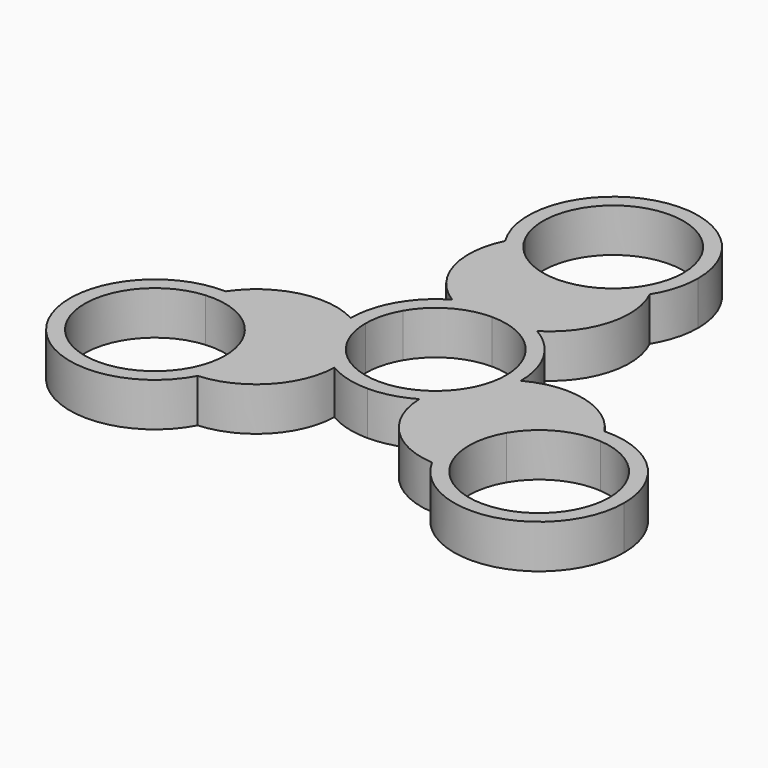
from build123d import *

# Parameters (mm, degrees)
F1_DEPTH = 5.9


with BuildPart() as f1:
    # F0 (on Top) → F1 (new body)
    with BuildSketch(Plane.XY):
        with BuildLine():
            Line((11.5, 0), (9.5, 0))
            ThreePointArc((9.5, 0), (9.1762953497, -2.4587809285), (8.227241336, -4.75))
            Line((8.227241336, -4.75), (9.9592921435, -5.75))
            ThreePointArc((9.9592921435, -5.75), (11.1081470023, -2.9764190187), (11.5, 0))
        make_face()
        with BuildLine():
            ThreePointArc((8.227241336, 4.75), (9.1762953497, 2.4587809285), (9.5, 0))
            Line((9.5, 0), (11.5, 0))
            ThreePointArc((11.5, 0), (11.1081470023, 2.9764190187), (9.9592921435, 5.75))
            Line((9.9592921435, 5.75), (8.227241336, 4.75))
        make_face()
        with BuildLine():
            ThreePointArc((0, 9.5), (4.75, 8.227241336), (8.227241336, 4.75))
            Line((8.227241336, 4.75), (9.9592921435, 5.75))
            ThreePointArc((9.9592921435, 5.75), (8.1317279836, 8.1317279836), (5.75, 9.9592921435))
            ThreePointArc((5.75, 9.9592921435), (2.9764190187, 11.1081470023), (0, 11.5))
            Line((0, 11.5), (0, 9.5))
        make_face()
        with BuildLine():
            Line((9.9592921435, -5.75), (8.227241336, -4.75))
            ThreePointArc((8.227241336, -4.75), (4.75, -8.227241336), (0, -9.5))
            Line((0, -9.5), (0, -11.5))
            ThreePointArc((0, -11.5), (2.9764190187, -11.1081470023), (5.75, -9.9592921435))
            ThreePointArc((5.75, -9.9592921435), (8.1317279836, -8.1317279836), (9.9592921435, -5.75))
        make_face()
        with BuildLine():
            Line((21.7644823154, 0), (11.5, 0))
            ThreePointArc((11.5, 0), (11.1081470023, -2.9764190187), (9.9592921435, -5.75))
            Line((9.9592921435, -5.75), (16.02146997, -9.25))
            ThreePointArc((16.02146997, -9.25), (20.0781480078, -5.1303927779), (25.6267837466, -3.5054491468))
            ThreePointArc((25.6267837466, -3.5054491468), (23.9098470955, -1.5167036662), (21.7644823154, 0))
        make_face()
        with BuildLine():
            ThreePointArc((21.7644823154, 0), (16.6322411577, 1.2934670156), (11.5, 0))
            Line((11.5, 0), (21.7644823154, 0))
        make_face()
        with BuildLine():
            ThreePointArc((-8.227241336, 4.75), (-4.75, 8.227241336), (0, 9.5))
            Line((0, 9.5), (0, 11.5))
            ThreePointArc((0, 11.5), (-2.9764190187, 11.1081470023), (-5.75, 9.9592921435))
            ThreePointArc((-5.75, 9.9592921435), (-8.1317279836, 8.1317279836), (-9.9592921435, 5.75))
            Line((-9.9592921435, 5.75), (-8.227241336, 4.75))
        make_face()
        with BuildLine():
            Line((0, -11.5), (0, -9.5))
            ThreePointArc((0, -9.5), (-4.75, -8.227241336), (-8.227241336, -4.75))
            Line((-8.227241336, -4.75), (-9.9592921435, -5.75))
            ThreePointArc((-9.9592921435, -5.75), (-8.1317279836, -8.1317279836), (-5.75, -9.9592921435))
            ThreePointArc((-5.75, -9.9592921435), (-2.9764190187, -11.1081470023), (0, -11.5))
        make_face()
        with BuildLine():
            Line((16.02146997, -9.25), (9.9592921435, -5.75))
            ThreePointArc((9.9592921435, -5.75), (8.1317279836, -8.1317279836), (5.75, -9.9592921435))
            ThreePointArc((5.75, -9.9592921435), (8.7759533757, -17.1498563505), (15.8491998862, -20.4407211685))
            ThreePointArc((15.8491998862, -20.4407211685), (14.4821244809, -14.8229898467), (16.02146997, -9.25))
        make_face()
        with BuildLine():
            Line((-9.9592921435, -5.75), (-8.227241336, -4.75))
            ThreePointArc((-8.227241336, -4.75), (-9.1762953497, -2.4587809285), (-9.5, 0))
            Line((-9.5, 0), (-11.5, 0))
            ThreePointArc((-11.5, 0), (-11.1081470023, -2.9764190187), (-9.9592921435, -5.75))
        make_face()
        with BuildLine():
            Line((-11.5, 0), (-9.5, 0))
            ThreePointArc((-9.5, 0), (-9.1762953497, 2.4587809285), (-8.227241336, 4.75))
            Line((-8.227241336, 4.75), (-9.9592921435, 5.75))
            ThreePointArc((-9.9592921435, 5.75), (-11.1081470023, 2.9764190187), (-11.5, 0))
        make_face()
        with BuildLine():
            Line((0, 18.5), (0, 11.5))
            ThreePointArc((0, 11.5), (2.9764190187, 11.1081470023), (5.75, 9.9592921435))
            ThreePointArc((5.75, 9.9592921435), (10.464234583, 16.1751267411), (9.7775838605, 23.9461703153))
            ThreePointArc((9.7775838605, 23.9461703153), (5.5960235268, 19.9533826246), (0, 18.5))
        make_face()
        with BuildLine():
            ThreePointArc((-5.75, 9.9592921435), (-2.9764190187, 11.1081470023), (0, 11.5))
            Line((0, 11.5), (0, 18.5))
            ThreePointArc((0, 18.5), (-5.5960235268, 19.9533826246), (-9.7775838605, 23.9461703153))
            ThreePointArc((-9.7775838605, 23.9461703153), (-10.464234583, 16.1751267411), (-5.75, 9.9592921435))
        make_face()
        with BuildLine():
            ThreePointArc((25.6267837466, -3.5054491468), (20.0781480078, -5.1303927779), (16.02146997, -9.25))
            Line((16.02146997, -9.25), (17.7535207776, -10.25))
            ThreePointArc((17.7535207776, -10.25), (21.5421151907, -6.6006897013), (26.6916116991, -5.5266324432))
            ThreePointArc((26.6916116991, -5.5266324432), (26.212648084, -4.4878813308), (25.6267837466, -3.5054491468))
        make_face()
        with BuildLine():
            Line((17.7535207776, -10.25), (16.02146997, -9.25))
            ThreePointArc((16.02146997, -9.25), (14.4821244809, -14.8229898467), (15.8491998862, -20.4407211685))
            ThreePointArc((15.8491998862, -20.4407211685), (16.9929432837, -20.4568784758), (18.1320099427, -20.3522975778))
            ThreePointArc((18.1320099427, -20.3522975778), (16.4874225591, -15.3556741558), (17.7535207776, -10.25))
        make_face()
        with BuildLine():
            Line((-16.02146997, -9.25), (-9.9592921435, -5.75))
            ThreePointArc((-9.9592921435, -5.75), (-11.1081470023, -2.9764190187), (-11.5, 0))
            Line((-11.5, 0), (-21.7644823154, 0))
            ThreePointArc((-21.7644823154, 0), (-23.9098470955, -1.5167036662), (-25.6267837466, -3.5054491468))
            ThreePointArc((-25.6267837466, -3.5054491468), (-20.0781480078, -5.1303927779), (-16.02146997, -9.25))
        make_face()
        with BuildLine():
            ThreePointArc((-5.75, -9.9592921435), (-8.1317279836, -8.1317279836), (-9.9592921435, -5.75))
            Line((-9.9592921435, -5.75), (-16.02146997, -9.25))
            ThreePointArc((-16.02146997, -9.25), (-14.8726151112, -12.0235809813), (-14.4807621135, -15))
            ThreePointArc((-14.4807621135, -15), (-14.8281174582, -17.8050877335), (-15.8491998862, -20.4407211685))
            ThreePointArc((-15.8491998862, -20.4407211685), (-8.7759533757, -17.1498563505), (-5.75, -9.9592921435))
        make_face()
        with BuildLine():
            Line((-21.7644823154, 0), (-11.5, 0))
            ThreePointArc((-11.5, 0), (-16.6322411577, 1.2934670156), (-21.7644823154, 0))
        make_face()
        with BuildLine():
            ThreePointArc((37.4807621135, -15), (33.9863616782, -6.7440702759), (25.6267837466, -3.5054491468))
            ThreePointArc((25.6267837466, -3.5054491468), (26.212648084, -4.4878813308), (26.6916116991, -5.5266324432))
            ThreePointArc((26.6916116991, -5.5266324432), (32.945066496, -8.5386948324), (35.4807621135, -15))
            ThreePointArc((35.4807621135, -15), (28.7813740446, -24.077806608), (18.1320099427, -20.3522975778))
            ThreePointArc((18.1320099427, -20.3522975778), (16.9929432837, -20.4568784758), (15.8491998862, -20.4407211685))
            ThreePointArc((15.8491998862, -20.4407211685), (28.785849847, -26.1526446553), (37.4807621135, -15))
        make_face()
        with BuildLine():
            ThreePointArc((-9.7775838605, 23.9461703153), (-5.5960235268, 19.9533826246), (0, 18.5))
            Line((0, 18.5), (0, 20.5))
            ThreePointArc((0, 20.5), (-5.0546926316, 21.956363857), (-8.5596017564, 25.8789300209))
            ThreePointArc((-8.5596017564, 25.8789300209), (-9.2197048003, 24.9447598066), (-9.7775838605, 23.9461703153))
        make_face()
        with BuildLine():
            Line((0, 20.5), (0, 18.5))
            ThreePointArc((0, 18.5), (5.5960235268, 19.9533826246), (9.7775838605, 23.9461703153))
            ThreePointArc((9.7775838605, 23.9461703153), (9.2197048003, 24.9447598066), (8.5596017564, 25.8789300209))
            ThreePointArc((8.5596017564, 25.8789300209), (5.0546926316, 21.956363857), (0, 20.5))
        make_face()
        with BuildLine():
            ThreePointArc((8.5596017564, 25.8789300209), (9.2197048003, 24.9447598066), (9.7775838605, 23.9461703153))
            ThreePointArc((9.7775838605, 23.9461703153), (11.0610174576, 26.8529549094), (11.5, 30))
            ThreePointArc((11.5, 30), (-3.1470450906, 41.0610174576), (-9.7775838605, 23.9461703153))
            ThreePointArc((-9.7775838605, 23.9461703153), (-9.2197048003, 24.9447598066), (-8.5596017564, 25.8789300209))
            ThreePointArc((-8.5596017564, 25.8789300209), (-2.1135022255, 39.2619170987), (9.5, 30))
            ThreePointArc((9.5, 30), (9.2619170987, 27.8864977745), (8.5596017564, 25.8789300209))
        make_face()
        with BuildLine():
            ThreePointArc((-14.4807621135, -15), (-14.8726151112, -12.0235809813), (-16.02146997, -9.25))
            Line((-16.02146997, -9.25), (-17.7535207776, -10.25))
            ThreePointArc((-17.7535207776, -10.25), (-16.8044667638, -12.5412190715), (-16.4807621135, -15))
            ThreePointArc((-16.4807621135, -15), (-16.9029555056, -17.8006119311), (-18.1320099427, -20.3522975778))
            ThreePointArc((-18.1320099427, -20.3522975778), (-16.9929432837, -20.4568784758), (-15.8491998862, -20.4407211685))
            ThreePointArc((-15.8491998862, -20.4407211685), (-14.8281174582, -17.8050877335), (-14.4807621135, -15))
        make_face()
        with BuildLine():
            Line((-17.7535207776, -10.25), (-16.02146997, -9.25))
            ThreePointArc((-16.02146997, -9.25), (-20.0781480078, -5.1303927779), (-25.6267837466, -3.5054491468))
            ThreePointArc((-25.6267837466, -3.5054491468), (-26.212648084, -4.4878813308), (-26.6916116991, -5.5266324432))
            ThreePointArc((-26.6916116991, -5.5266324432), (-21.5421151907, -6.6006897013), (-17.7535207776, -10.25))
        make_face()
        with BuildLine():
            ThreePointArc((-25.6267837466, -3.5054491468), (-35.9400542571, -20.75), (-15.8491998862, -20.4407211685))
            ThreePointArc((-15.8491998862, -20.4407211685), (-16.9929432837, -20.4568784758), (-18.1320099427, -20.3522975778))
            ThreePointArc((-18.1320099427, -20.3522975778), (-34.2080034495, -19.75), (-26.6916116991, -5.5266324432))
            ThreePointArc((-26.6916116991, -5.5266324432), (-26.212648084, -4.4878813308), (-25.6267837466, -3.5054491468))
        make_face()
    extrude(amount=F1_DEPTH)


solid = f1.part
